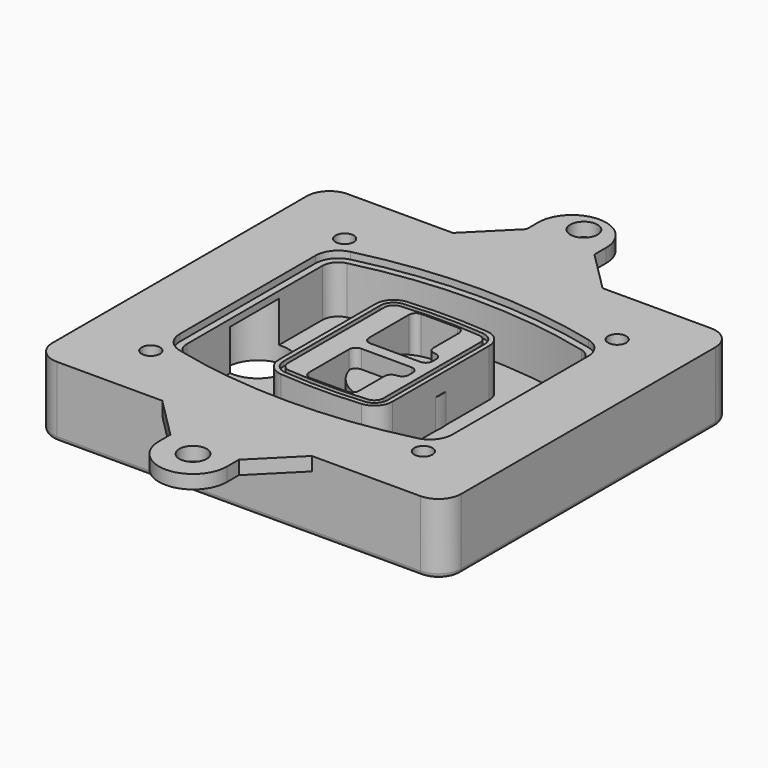
from build123d import *

# Parameters (mm, degrees)
F0_R      = 4
F1_DEPTH  = 25
F2_DEPTH  = 3
F3_DEPTH  = 18
F5_DEPTH  = 21
F6_DEPTH  = 2
F8_DEPTH  = 20
F9_DEPTH  = 16
F10_DEPTH = 25
F7_R      = 6
F7_R_2    = 4
F11_DEPTH = 6
F13_DEPTH = 9
F15_R     = 2
F16_R     = 4
F16_R_2   = 6
F17_DEPTH = 6


# Not quite as in the source:
# - a feature of the source that left no trace in its solid (it failed there, or was rolled back) is left out
# - a feature names something its author has since deleted; it is built from what else it names


with BuildPart() as f1:
    # F0 (on Top) → F1 (new body)
    with BuildSketch(Plane.XY):
        with BuildLine():
            ThreePointArc((-90, -70), (-87.0710678119, -77.0710678119), (-80, -80))
            Line((-80, -80), (80, -80))
            ThreePointArc((80, -80), (87.0710678119, -77.0710678119), (90, -70))
            Line((90, -70), (90, 70))
            ThreePointArc((90, 70), (87.0710678119, 77.0710678119), (80, 80))
            Line((80, 80), (-80, 80))
            ThreePointArc((-80, 80), (-87.0710678119, 77.0710678119), (-90, 70))
            Line((-90, 70), (-90, -70))
        make_face()
        with Locations((-60, -53.3333333333)):
            Circle(F0_R, mode=Mode.SUBTRACT)
        with Locations((60, -53.3333333333)):
            Circle(F0_R, mode=Mode.SUBTRACT)
        with Locations((-60, 53.3333333333)):
            Circle(F0_R, mode=Mode.SUBTRACT)
        with BuildLine():
            ThreePointArc((-64, 37.2990447398), (-61.0143011354, 45.9411029726), (-53.3306899286, 50.8970778549))
            ThreePointArc((-53.3306899286, 50.8970778549), (0, 57.3333333333), (53.3306899286, 50.8970778549))
            ThreePointArc((53.3306899286, 50.8970778549), (61.0143011354, 45.9411029726), (64, 37.2990447398))
            Line((64, 37.2990447398), (64, -37.2990447398))
            ThreePointArc((64, -37.2990447398), (61.0143011354, -45.9411029726), (53.3306899286, -50.8970778549))
            ThreePointArc((53.3306899286, -50.8970778549), (0, -57.3333333333), (-53.3306899286, -50.8970778549))
            ThreePointArc((-53.3306899286, -50.8970778549), (-61.0143011354, -45.9411029726), (-64, -37.2990447398))
            Line((-64, -37.2990447398), (-64, 37.2990447398))
        make_face(mode=Mode.SUBTRACT)
        with Locations((60, 53.3333333333)):
            Circle(F0_R, mode=Mode.SUBTRACT)
        with BuildLine():
            ThreePointArc((53.3306899286, 50.8970778549), (0, 57.3333333333), (-53.3306899286, 50.8970778549))
            ThreePointArc((-53.3306899286, 50.8970778549), (-61.0143011354, 45.9411029726), (-64, 37.2990447398))
            Line((-64, 37.2990447398), (-64, -37.2990447398))
            ThreePointArc((-64, -37.2990447398), (-61.0143011354, -45.9411029726), (-53.3306899286, -50.8970778549))
            ThreePointArc((-53.3306899286, -50.8970778549), (0, -57.3333333333), (53.3306899286, -50.8970778549))
            ThreePointArc((53.3306899286, -50.8970778549), (61.0143011354, -45.9411029726), (64, -37.2990447398))
            Line((64, -37.2990447398), (64, 37.2990447398))
            ThreePointArc((64, 37.2990447398), (61.0143011354, 45.9411029726), (53.3306899286, 50.8970778549))
        make_face()
        with BuildLine():
            Line((-60, -37.2990447398), (-60, 37.2990447398))
            ThreePointArc((-60, 37.2990447398), (-57.8673579538, 43.4719434775), (-52.3790642347, 47.0119255363))
            ThreePointArc((-52.3790642347, 47.0119255363), (0, 53.3333333333), (52.3790642347, 47.0119255363))
            ThreePointArc((52.3790642347, 47.0119255363), (57.8673579538, 43.4719434775), (60, 37.2990447398))
            Line((60, 37.2990447398), (60, -37.2990447398))
            ThreePointArc((60, -37.2990447398), (57.8673579538, -43.4719434775), (52.3790642347, -47.0119255363))
            ThreePointArc((52.3790642347, -47.0119255363), (0, -53.3333333333), (-52.3790642347, -47.0119255363))
            ThreePointArc((-52.3790642347, -47.0119255363), (-57.8673579538, -43.4719434775), (-60, -37.2990447398))
        make_face(mode=Mode.SUBTRACT)
        with BuildLine():
            ThreePointArc((-52.3790642347, 47.0119255363), (-57.8673579538, 43.4719434775), (-60, 37.2990447398))
            Line((-60, 37.2990447398), (-60, -37.2990447398))
            ThreePointArc((-60, -37.2990447398), (-57.8673579538, -43.4719434775), (-52.3790642347, -47.0119255363))
            ThreePointArc((-52.3790642347, -47.0119255363), (0, -53.3333333333), (52.3790642347, -47.0119255363))
            ThreePointArc((52.3790642347, -47.0119255363), (57.8673579538, -43.4719434775), (60, -37.2990447398))
            Line((60, -37.2990447398), (60, 37.2990447398))
            ThreePointArc((60, 37.2990447398), (57.8673579538, 43.4719434775), (52.3790642347, 47.0119255363))
            ThreePointArc((52.3790642347, 47.0119255363), (0, 53.3333333333), (-52.3790642347, 47.0119255363))
        make_face()
        with BuildLine():
            ThreePointArc((51.6653449643, 44.0980612973), (55.5071505677, 41.6200738562), (57, 37.2990447398))
            Line((57, 37.2990447398), (57, -37.2990447398))
            ThreePointArc((57, -37.2990447398), (55.5071505677, -41.6200738562), (51.6653449643, -44.0980612973))
            ThreePointArc((51.6653449643, -44.0980612973), (0, -50.3333333333), (-51.6653449643, -44.0980612973))
            ThreePointArc((-51.6653449643, -44.0980612973), (-55.5071505677, -41.6200738562), (-57, -37.2990447398))
            Line((-57, -37.2990447398), (-57, 37.2990447398))
            ThreePointArc((-57, 37.2990447398), (-55.5071505677, 41.6200738562), (-51.6653449643, 44.0980612973))
            ThreePointArc((-51.6653449643, 44.0980612973), (0, 50.3333333333), (51.6653449643, 44.0980612973))
        make_face(mode=Mode.SUBTRACT)
        with BuildLine():
            Line((57, -37.2990447398), (57, 37.2990447398))
            ThreePointArc((57, 37.2990447398), (55.5071505677, 41.6200738562), (51.6653449643, 44.0980612973))
            ThreePointArc((51.6653449643, 44.0980612973), (0, 50.3333333333), (-51.6653449643, 44.0980612973))
            ThreePointArc((-51.6653449643, 44.0980612973), (-55.5071505677, 41.6200738562), (-57, 37.2990447398))
            Line((-57, 37.2990447398), (-57, -37.2990447398))
            ThreePointArc((-57, -37.2990447398), (-55.5071505677, -41.6200738562), (-51.6653449643, -44.0980612973))
            ThreePointArc((-51.6653449643, -44.0980612973), (0, -50.3333333333), (51.6653449643, -44.0980612973))
            ThreePointArc((51.6653449643, -44.0980612973), (55.5071505677, -41.6200738562), (57, -37.2990447398))
        make_face()
    extrude(amount=-F1_DEPTH)

    # F0 (on Top) → F2 (join)
    with BuildSketch(Plane.XY):
        with BuildLine():
            ThreePointArc((-52.3790642347, 47.0119255363), (-57.8673579538, 43.4719434775), (-60, 37.2990447398))
            Line((-60, 37.2990447398), (-60, -37.2990447398))
            ThreePointArc((-60, -37.2990447398), (-57.8673579538, -43.4719434775), (-52.3790642347, -47.0119255363))
            ThreePointArc((-52.3790642347, -47.0119255363), (0, -53.3333333333), (52.3790642347, -47.0119255363))
            ThreePointArc((52.3790642347, -47.0119255363), (57.8673579538, -43.4719434775), (60, -37.2990447398))
            Line((60, -37.2990447398), (60, 37.2990447398))
            ThreePointArc((60, 37.2990447398), (57.8673579538, 43.4719434775), (52.3790642347, 47.0119255363))
            ThreePointArc((52.3790642347, 47.0119255363), (0, 53.3333333333), (-52.3790642347, 47.0119255363))
        make_face()
        with BuildLine():
            ThreePointArc((51.6653449643, 44.0980612973), (55.5071505677, 41.6200738562), (57, 37.2990447398))
            Line((57, 37.2990447398), (57, -37.2990447398))
            ThreePointArc((57, -37.2990447398), (55.5071505677, -41.6200738562), (51.6653449643, -44.0980612973))
            ThreePointArc((51.6653449643, -44.0980612973), (0, -50.3333333333), (-51.6653449643, -44.0980612973))
            ThreePointArc((-51.6653449643, -44.0980612973), (-55.5071505677, -41.6200738562), (-57, -37.2990447398))
            Line((-57, -37.2990447398), (-57, 37.2990447398))
            ThreePointArc((-57, 37.2990447398), (-55.5071505677, 41.6200738562), (-51.6653449643, 44.0980612973))
            ThreePointArc((-51.6653449643, 44.0980612973), (0, 50.3333333333), (51.6653449643, 44.0980612973))
        make_face(mode=Mode.SUBTRACT)
    extrude(amount=F2_DEPTH)

    # F0 (on Top) → F3 (cut)
    with BuildSketch(Plane.XY):
        with BuildLine():
            Line((57, -37.2990447398), (57, 37.2990447398))
            ThreePointArc((57, 37.2990447398), (55.5071505677, 41.6200738562), (51.6653449643, 44.0980612973))
            ThreePointArc((51.6653449643, 44.0980612973), (0, 50.3333333333), (-51.6653449643, 44.0980612973))
            ThreePointArc((-51.6653449643, 44.0980612973), (-55.5071505677, 41.6200738562), (-57, 37.2990447398))
            Line((-57, 37.2990447398), (-57, -37.2990447398))
            ThreePointArc((-57, -37.2990447398), (-55.5071505677, -41.6200738562), (-51.6653449643, -44.0980612973))
            ThreePointArc((-51.6653449643, -44.0980612973), (0, -50.3333333333), (51.6653449643, -44.0980612973))
            ThreePointArc((51.6653449643, -44.0980612973), (55.5071505677, -41.6200738562), (57, -37.2990447398))
        make_face()
    extrude(amount=-F3_DEPTH, mode=Mode.SUBTRACT)

    # F4 (on face) → F5 (join, through all)
    with BuildSketch(Plane.XY.offset(3)):
        with BuildLine():
            ThreePointArc((-25, -26.587695628), (-22.8992979869, -31.9912392117), (-17.7004291845, -34.5569740744))
            ThreePointArc((-17.7004291845, -34.5569740744), (0, -35.3333333333), (17.7004291845, -34.5569740744))
            ThreePointArc((17.7004291845, -34.5569740744), (22.8992979869, -31.9912392117), (25, -26.587695628))
            Line((25, -26.587695628), (25, 26.587695628))
            ThreePointArc((25, 26.587695628), (22.8992979869, 31.9912392117), (17.7004291845, 34.5569740744))
            ThreePointArc((17.7004291845, 34.5569740744), (0, 35.3333333333), (-17.7004291845, 34.5569740744))
            ThreePointArc((-17.7004291845, 34.5569740744), (-22.8992979869, 31.9912392117), (-25, 26.587695628))
            Line((-25, 26.587695628), (-25, -26.587695628))
        make_face()
        with BuildLine():
            ThreePointArc((17.5253218884, 32.5646544628), (21.4244734902, 30.6403533158), (23, 26.587695628))
            Line((23, 26.587695628), (23, -26.587695628))
            ThreePointArc((23, -26.587695628), (21.4244734902, -30.6403533158), (17.5253218884, -32.5646544628))
            ThreePointArc((17.5253218884, -32.5646544628), (0, -33.3333333333), (-17.5253218884, -32.5646544628))
            ThreePointArc((-17.5253218884, -32.5646544628), (-21.4244734902, -30.6403533158), (-23, -26.587695628))
            Line((-23, -26.587695628), (-23, 26.587695628))
            ThreePointArc((-23, 26.587695628), (-21.4244734902, 30.6403533158), (-17.5253218884, 32.5646544628))
            ThreePointArc((-17.5253218884, 32.5646544628), (0, 33.3333333333), (17.5253218884, 32.5646544628))
        make_face(mode=Mode.SUBTRACT)
        with BuildLine():
            Line((23, -26.587695628), (23, 26.587695628))
            ThreePointArc((23, 26.587695628), (21.4244734902, 30.6403533158), (17.5253218884, 32.5646544628))
            ThreePointArc((17.5253218884, 32.5646544628), (0, 33.3333333333), (-17.5253218884, 32.5646544628))
            ThreePointArc((-17.5253218884, 32.5646544628), (-21.4244734902, 30.6403533158), (-23, 26.587695628))
            Line((-23, 26.587695628), (-23, -26.587695628))
            ThreePointArc((-23, -26.587695628), (-21.4244734902, -30.6403533158), (-17.5253218884, -32.5646544628))
            ThreePointArc((-17.5253218884, -32.5646544628), (0, -33.3333333333), (17.5253218884, -32.5646544628))
            ThreePointArc((17.5253218884, -32.5646544628), (21.4244734902, -30.6403533158), (23, -26.587695628))
        make_face()
        with BuildLine():
            ThreePointArc((17.3502145923, 30.5723348512), (19.9496489934, 29.2894674198), (21, 26.587695628))
            Line((21, 26.587695628), (21, -26.587695628))
            ThreePointArc((21, -26.587695628), (19.9496489934, -29.2894674198), (17.3502145923, -30.5723348512))
            ThreePointArc((17.3502145923, -30.5723348512), (0, -31.3333333333), (-17.3502145923, -30.5723348512))
            ThreePointArc((-17.3502145923, -30.5723348512), (-19.9496489934, -29.2894674198), (-21, -26.587695628))
            Line((-21, -26.587695628), (-21, 26.587695628))
            ThreePointArc((-21, 26.587695628), (-19.9496489934, 29.2894674198), (-17.3502145923, 30.5723348512))
            ThreePointArc((-17.3502145923, 30.5723348512), (0, 31.3333333333), (17.3502145923, 30.5723348512))
        make_face(mode=Mode.SUBTRACT)
        with BuildLine():
            Line((21, -26.587695628), (21, 26.587695628))
            ThreePointArc((21, 26.587695628), (19.9496489934, 29.2894674198), (17.3502145923, 30.5723348512))
            ThreePointArc((17.3502145923, 30.5723348512), (0, 31.3333333333), (-17.3502145923, 30.5723348512))
            ThreePointArc((-17.3502145923, 30.5723348512), (-19.9496489934, 29.2894674198), (-21, 26.587695628))
            Line((-21, 26.587695628), (-21, -26.587695628))
            ThreePointArc((-21, -26.587695628), (-19.9496489934, -29.2894674198), (-17.3502145923, -30.5723348512))
            ThreePointArc((-17.3502145923, -30.5723348512), (0, -31.3333333333), (17.3502145923, -30.5723348512))
            ThreePointArc((17.3502145923, -30.5723348512), (19.9496489934, -29.2894674198), (21, -26.587695628))
        make_face()
        with BuildLine():
            Line((-8, -2.5), (14, -2.5))
            ThreePointArc((14, -2.5), (16.1213203436, -3.3786796564), (17, -5.5))
            Line((17, -5.5), (17, -7.5))
            ThreePointArc((17, -7.5), (16.1213203436, -9.6213203436), (14, -10.5))
            ThreePointArc((14, -10.5), (11.8786796564, -11.3786796564), (11, -13.5))
            Line((11, -13.5), (11, -27.5))
            ThreePointArc((11, -27.5), (10.1213203436, -29.6213203436), (8, -30.5))
            Line((8, -30.5), (-8, -30.5))
            ThreePointArc((-8, -30.5), (-10.1213203436, -29.6213203436), (-11, -27.5))
            Line((-11, -27.5), (-11, -5.5))
            ThreePointArc((-11, -5.5), (-10.1213203436, -3.3786796564), (-8, -2.5))
        make_face(mode=Mode.SUBTRACT)
        with BuildLine():
            ThreePointArc((-8, 2.5), (-10.1213203436, 3.3786796564), (-11, 5.5))
            Line((-11, 5.5), (-11, 27.5))
            ThreePointArc((-11, 27.5), (-10.1213203436, 29.6213203436), (-8, 30.5))
            Line((-8, 30.5), (8, 30.5))
            ThreePointArc((8, 30.5), (10.1213203436, 29.6213203436), (11, 27.5))
            Line((11, 27.5), (11, 13.5))
            ThreePointArc((11, 13.5), (11.8786796564, 11.3786796564), (14, 10.5))
            ThreePointArc((14, 10.5), (16.1213203436, 9.6213203436), (17, 7.5))
            Line((17, 7.5), (17, 5.5))
            ThreePointArc((17, 5.5), (16.1213203436, 3.3786796564), (14, 2.5))
            Line((14, 2.5), (-8, 2.5))
        make_face(mode=Mode.SUBTRACT)
    extrude(amount=-F5_DEPTH)

    # F4 (on face) → F6 (cut)
    with BuildSketch(Plane.XY.offset(3)):
        with BuildLine():
            Line((23, -26.587695628), (23, 26.587695628))
            ThreePointArc((23, 26.587695628), (21.4244734902, 30.6403533158), (17.5253218884, 32.5646544628))
            ThreePointArc((17.5253218884, 32.5646544628), (0, 33.3333333333), (-17.5253218884, 32.5646544628))
            ThreePointArc((-17.5253218884, 32.5646544628), (-21.4244734902, 30.6403533158), (-23, 26.587695628))
            Line((-23, 26.587695628), (-23, -26.587695628))
            ThreePointArc((-23, -26.587695628), (-21.4244734902, -30.6403533158), (-17.5253218884, -32.5646544628))
            ThreePointArc((-17.5253218884, -32.5646544628), (0, -33.3333333333), (17.5253218884, -32.5646544628))
            ThreePointArc((17.5253218884, -32.5646544628), (21.4244734902, -30.6403533158), (23, -26.587695628))
        make_face()
        with BuildLine():
            ThreePointArc((17.3502145923, 30.5723348512), (19.9496489934, 29.2894674198), (21, 26.587695628))
            Line((21, 26.587695628), (21, -26.587695628))
            ThreePointArc((21, -26.587695628), (19.9496489934, -29.2894674198), (17.3502145923, -30.5723348512))
            ThreePointArc((17.3502145923, -30.5723348512), (0, -31.3333333333), (-17.3502145923, -30.5723348512))
            ThreePointArc((-17.3502145923, -30.5723348512), (-19.9496489934, -29.2894674198), (-21, -26.587695628))
            Line((-21, -26.587695628), (-21, 26.587695628))
            ThreePointArc((-21, 26.587695628), (-19.9496489934, 29.2894674198), (-17.3502145923, 30.5723348512))
            ThreePointArc((-17.3502145923, 30.5723348512), (0, 31.3333333333), (17.3502145923, 30.5723348512))
        make_face(mode=Mode.SUBTRACT)
    extrude(amount=-F6_DEPTH, mode=Mode.SUBTRACT)

    # F7 (on face) → F8 (join)
    with BuildSketch(Plane(origin=(0, 0, -25), x_dir=(1, 0, 0), z_dir=(0, 0, -1))):
        with BuildLine():
            ThreePointArc((-6.71157564, 0), (6.7567035675, 13.4682792075), (20.224982775, 0))
            Line((20.224982775, 0), (25.224982775, 0))
            ThreePointArc((25.224982775, 0), (6.7567035675, 18.4682792075), (-11.71157564, 0))
            Line((-11.71157564, 0), (-6.71157564, 0))
        make_face()
        with BuildLine():
            Line((-6.71157564, 0), (20.224982775, 0))
            ThreePointArc((20.224982775, 0), (6.7567035675, 13.4682792075), (-6.71157564, 0))
        make_face()
        with BuildLine():
            ThreePointArc((-6.71157564, 0), (6.7567035675, -13.4682792075), (20.224982775, 0))
            Line((20.224982775, 0), (-6.71157564, 0))
        make_face()
        with BuildLine():
            Line((25.224982775, 0), (20.224982775, 0))
            ThreePointArc((20.224982775, 0), (6.7567035675, -13.4682792075), (-6.71157564, 0))
            Line((-6.71157564, 0), (-11.71157564, 0))
            ThreePointArc((-11.71157564, 0), (6.7567035675, -18.4682792075), (25.224982775, 0))
        make_face()
    extrude(amount=-F8_DEPTH)

    # F7 (on face) → F9 (cut)
    with BuildSketch(Plane(origin=(0, 0, -25), x_dir=(1, 0, 0), z_dir=(0, 0, -1))):
        with BuildLine():
            Line((-6.71157564, 0), (20.224982775, 0))
            ThreePointArc((20.224982775, 0), (6.7567035675, 13.4682792075), (-6.71157564, 0))
        make_face()
        with BuildLine():
            ThreePointArc((-6.71157564, 0), (6.7567035675, -13.4682792075), (20.224982775, 0))
            Line((20.224982775, 0), (-6.71157564, 0))
        make_face()
    extrude(amount=-F9_DEPTH, mode=Mode.SUBTRACT)

    # F7 (on face) → F10 (cut)
    with BuildSketch(Plane(origin=(0, 0, -25), x_dir=(1, 0, 0), z_dir=(0, 0, -1))):
        with BuildLine():
            Line((-69.0318229325, 0), (-42.0952645175, 0))
            ThreePointArc((-42.0952645175, 0), (-55.563543725, 13.4682792075), (-69.0318229325, 0))
        make_face()
        with BuildLine():
            ThreePointArc((-69.0318229325, 0), (-55.563543725, -13.4682792075), (-42.0952645175, 0))
            Line((-42.0952645175, 0), (-69.0318229325, 0))
        make_face()
    extrude(amount=-F10_DEPTH, mode=Mode.SUBTRACT)

    # F7 (on face) → F11 (cut)
    with BuildSketch(Plane(origin=(0, 0, -25), x_dir=(1, 0, 0), z_dir=(0, 0, -1))):
        with Locations((60, -53.3333333333)):
            Circle(F7_R)
        with Locations((60, -53.3333333333)):
            Circle(F7_R_2, mode=Mode.SUBTRACT)
        with Locations((-60, -53.3333333333)):
            Circle(F7_R)
        with Locations((-60, -53.3333333333)):
            Circle(F7_R_2, mode=Mode.SUBTRACT)
        with Locations((-60, 53.3333333333)):
            Circle(F7_R)
        with Locations((-60, 53.3333333333)):
            Circle(F7_R_2, mode=Mode.SUBTRACT)
        with Locations((60, 53.3333333333)):
            Circle(F7_R)
        with Locations((60, 53.3333333333)):
            Circle(F7_R_2, mode=Mode.SUBTRACT)
    extrude(amount=-F11_DEPTH, mode=Mode.SUBTRACT)

    # F12 (on face) → F13 (cut, through all)
    with BuildSketch(Plane(origin=(0, 0, -9), x_dir=(1, 0, 0), z_dir=(0, 0, -1))):
        with BuildLine():
            ThreePointArc((20.224982775, 0), (20.1663399806, 1.2554664788), (19.9909222755, 2.5))
            Line((19.9909222755, 2.5), (14, 2.5))
            ThreePointArc((14, 2.5), (16.1213203436, 3.3786796564), (17, 5.5))
            Line((17, 5.5), (17, 7.5))
            ThreePointArc((17, 7.5), (16.1213203436, 9.6213203436), (14, 10.5))
            ThreePointArc((14, 10.5), (12.1627255951, 11.1284134507), (11.0951631559, 12.750384826))
            ThreePointArc((11.0951631559, 12.750384826), (11.0476113807, 12.7664660322), (11, 12.7823698976))
            Line((11, 12.7823698976), (11, -12.7823698976))
            ThreePointArc((11, -12.7823698976), (11.0476113807, -12.7664660322), (11.0951631559, -12.750384826))
            ThreePointArc((11.0951631559, -12.750384826), (12.1627255951, -11.1284134507), (14, -10.5))
            ThreePointArc((14, -10.5), (16.1213203436, -9.6213203436), (17, -7.5))
            Line((17, -7.5), (17, -5.5))
            ThreePointArc((17, -5.5), (16.1213203436, -3.3786796564), (14, -2.5))
            Line((14, -2.5), (19.9909222755, -2.5))
            ThreePointArc((19.9909222755, -2.5), (20.1663399806, -1.2554664788), (20.224982775, 0))
        make_face()
    extrude(amount=F13_DEPTH, mode=Mode.SUBTRACT)

    # F15
    f15_edges = [f1.edges().sort_by_distance(p)[0] for p in [
        (0, -80, -25),
        (-87.071068, -77.071068, -25),
        (-90, 0, -25),
        (-87.071068, 77.071068, -25),
        (87.071068, -77.071068, -25),
        (0, 80, -25),
        (90, 0, -25),
        (87.071068, 77.071068, -25),
    ]]
    fillet(f15_edges, radius=F15_R)

    # F16 (on face) → F17 (join)
    with BuildSketch(Plane.XY):
        with BuildLine():
            Line((-33.6357802153, 80), (-80, 80))
            ThreePointArc((-80, 80), (-87.0710678119, 77.0710678119), (-90, 70))
            Line((-90, 70), (-90, -70))
            ThreePointArc((-90, -70), (-87.0710678119, -77.0710678119), (-80, -80))
            Line((-80, -80), (-33.6357802153, -80))
            Line((-33.6357802153, -80), (32.2245204587, -80))
            Line((32.2245204587, -80), (80, -80))
            ThreePointArc((80, -80), (87.0710678119, -77.0710678119), (90, -70))
            Line((90, -70), (90, 70))
            ThreePointArc((90, 70), (87.0710678119, 77.0710678119), (80, 80))
            Line((80, 80), (32.2245204587, 80))
            Line((32.2245204587, 80), (-33.6357802153, 80))
        make_face()
        with Locations((-60, -53.3333333333)):
            Circle(F16_R, mode=Mode.SUBTRACT)
        with Locations((60, -53.3333333333)):
            Circle(F16_R, mode=Mode.SUBTRACT)
        with Locations((-60, 53.3333333333)):
            Circle(F16_R, mode=Mode.SUBTRACT)
        with BuildLine():
            ThreePointArc((-52.3790642347, 47.0119255363), (0, 53.3333333333), (52.3790642347, 47.0119255363))
            ThreePointArc((52.3790642347, 47.0119255363), (57.8673579538, 43.4719434775), (60, 37.2990447398))
            Line((60, 37.2990447398), (60, -37.2990447398))
            ThreePointArc((60, -37.2990447398), (57.8673579538, -43.4719434775), (52.3790642347, -47.0119255363))
            ThreePointArc((52.3790642347, -47.0119255363), (0, -53.3333333333), (-52.3790642347, -47.0119255363))
            ThreePointArc((-52.3790642347, -47.0119255363), (-57.8673579538, -43.4719434775), (-60, -37.2990447398))
            Line((-60, -37.2990447398), (-60, 37.2990447398))
            ThreePointArc((-60, 37.2990447398), (-57.8673579538, 43.4719434775), (-52.3790642347, 47.0119255363))
        make_face(mode=Mode.SUBTRACT)
        with Locations((60, 53.3333333333)):
            Circle(F16_R, mode=Mode.SUBTRACT)
        with BuildLine():
            Line((-15.6357802153, 98), (-33.6357802153, 80))
            Line((-33.6357802153, 80), (32.2245204587, 80))
            Line((32.2245204587, 80), (14.3641984707, 97.8603219879))
            Line((14.3641984707, 97.8603219879), (14.3641984707, 104.3061713768))
            ThreePointArc((14.3641984707, 104.3061713768), (-0.6484449104, 119.3061660483), (-15.6357802153, 104.2808846236))
            Line((-15.6357802153, 104.2808846236), (-15.6357802153, 98))
        make_face()
        with Locations((0, 110)):
            Circle(F16_R_2, mode=Mode.SUBTRACT)
        with BuildLine():
            Line((32.2245204587, -80), (-33.6357802153, -80))
            Line((-33.6357802153, -80), (-15.6357802153, -98))
            Line((-15.6357802153, -98), (-15.6357802153, -104.2808846236))
            ThreePointArc((-15.6357802153, -104.2808846236), (-0.6484449104, -119.3061660483), (14.3641984707, -104.3061713768))
            Line((14.3641984707, -104.3061713768), (14.3641984707, -97.8603219879))
            Line((14.3641984707, -97.8603219879), (32.2245204587, -80))
        make_face()
        with Locations((-0.6358015293, -104.3061713768)):
            Circle(F16_R_2, mode=Mode.SUBTRACT)
    extrude(amount=F17_DEPTH)


solid = f1.part
